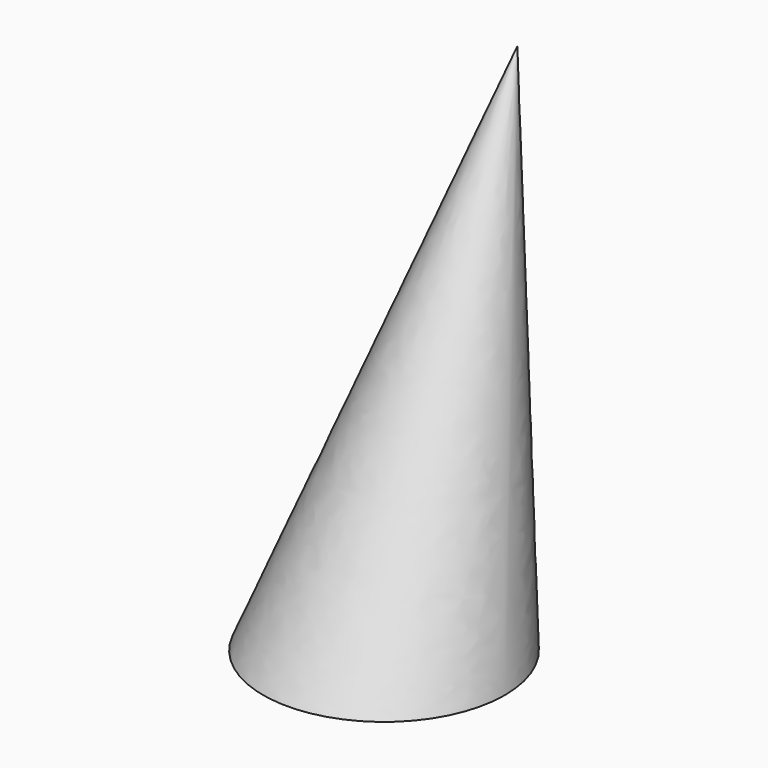
from build123d import *

# Parameters (mm, degrees)
F0_R = 19.8518026118


with BuildPart() as f3:
    # F0 (on Top) → F3 section 0
    with BuildSketch(Plane.XY, mode=Mode.PRIVATE) as f3_s0:
        Circle(F0_R)
    loft([Vertex(0, 27.3627266288, 76.2), f3_s0.sketch])


solid = f3.part
